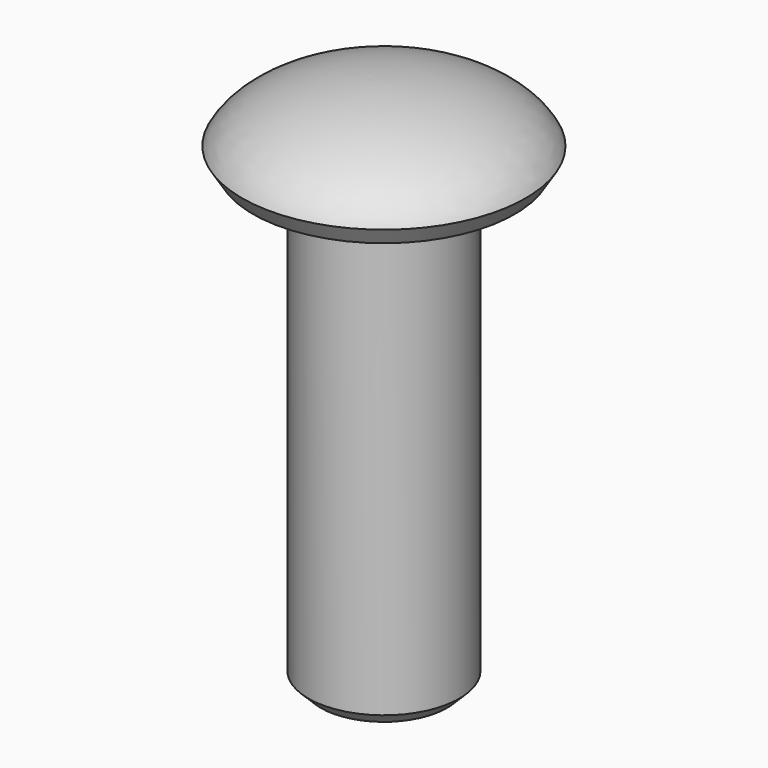
from build123d import *


# Not quite as in the source:
# - a fillet or chamfer that OpenCascade refuses, or shapes differently, is made with other operations: its cross-section is extruded or revolved along the edge and cut away or added


with BuildPart() as f1:
    # F0 (on Front) → F1 (revolve)
    with BuildSketch(Plane.XZ):
        with BuildLine():
            Line((0, 0), (0, 1.524))
            add(Edge.make_bspline(
                [(0, 1.524), (-3.048, 1.524), (-3.048, 0)],
                knots=[4.7123889804, 4.7123889804, 4.7123889804, 6.2831853072, 6.2831853072, 6.2831853072], degree=2, weights=[1, 0.7071067812, 1]))
            Line((-3.048, 0), (-1.5748, 0))
            Line((-1.5748, 0), (-1.5748, -9.525))
            Line((-1.5748, -9.525), (0, -9.525))
            Line((0, -9.525), (0, 0))
        make_face()
    revolve(axis=Axis((0, 0, -4.7625), (0, 0, -1)))

    # F2: chamfer of 0.254 on 2 edges, made by hand

    # F2_s1 → F2_t2 (revolve, cut)
    with BuildSketch(Plane.XZ):
        with BuildLine():
            Line((-2.9637200902, 0.3755062705), (-2.7254667291, -0.0086341425))
            Line((-2.7254667291, -0.0086341425), (-2.7254667291, -0.0137141425))
            ThreePointArc((-2.7254667291, -0.0137141425), (-2.8867333645, -0.00508), (-3.048, -0.00508))
            Line((-3.048, -0.00508), (-3.05308, 0))
            ThreePointArc((-3.05308, 0), (-3.0285671626, 0.1935290139), (-2.9682709531, 0.377763713))
            Line((-2.9682709531, 0.377763713), (-2.9637200902, 0.3755062705))
        make_face()
    revolve(axis=Axis((0, 0, 0), (0, 0, -1)), mode=Mode.SUBTRACT)

    # F2_s3 → F2_t4 (revolve, cut)
    with BuildSketch(Plane.XZ):
        with BuildLine():
            Line((-1.5819842049, -9.2638157951), (-1.3136157951, -9.5321842049))
            Line((-1.3136157951, -9.5321842049), (-1.3136157951, -9.5372642049))
            ThreePointArc((-1.3136157951, -9.5372642049), (-1.4442078976, -9.53008), (-1.5748, -9.53008))
            Line((-1.5748, -9.53008), (-1.57988, -9.525))
            ThreePointArc((-1.57988, -9.525), (-1.57988, -9.3944078976), (-1.5870642049, -9.2638157951))
            Line((-1.5870642049, -9.2638157951), (-1.5819842049, -9.2638157951))
        make_face()
    revolve(axis=Axis((0, 0, -9.525), (0, 0, -1)), mode=Mode.SUBTRACT)


solid = f1.part
